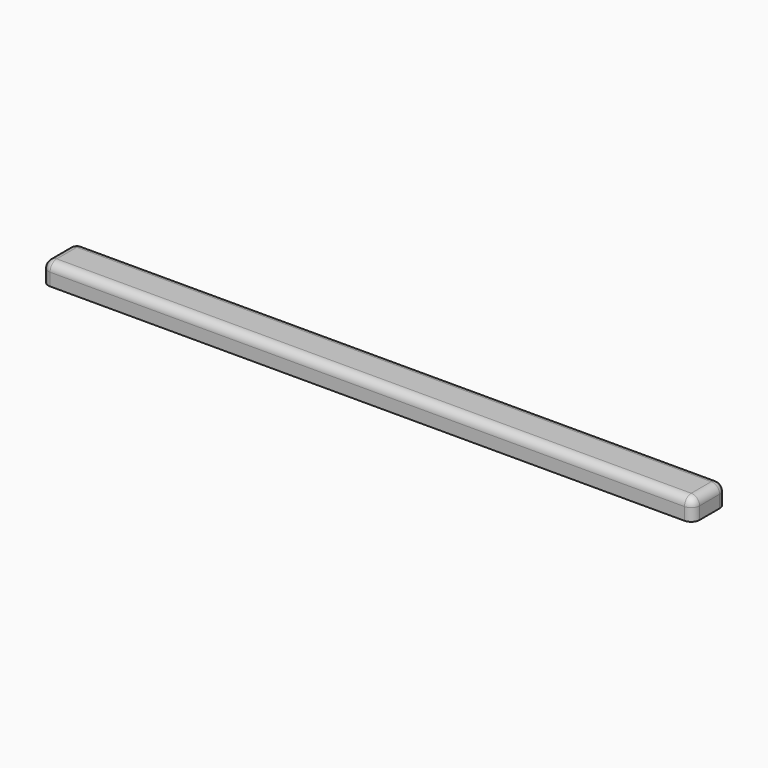
from build123d import *

# Parameters (mm, degrees)
F0_W         = 156
F0_H         = 10
F1_DEPTH     = 5
F2_R         = 2
F3_T1_DEPTH  = 8
F3_S5_W      = 2
F3_S5_H      = 2
F3_T6_DEPTH  = 2
F3_S11_W     = 2
F3_S11_H     = 2
F3_T12_DEPTH = 2
F3_S17_W     = 2
F3_S17_H     = 2
F3_T18_DEPTH = 2
F3_S23_W     = 2
F3_S23_H     = 2
F3_T24_DEPTH = 2


# Not quite as in the source:
# - a fillet or chamfer that OpenCascade refuses, or shapes differently, is made with other operations: its cross-section is extruded or revolved along the edge and cut away or added


with BuildPart() as f1:
    # F0 (on Top) → F1 (new body)
    with BuildSketch(Plane.XY):
        with Locations((-78, 5)):
            Rectangle(F0_W, F0_H)
    extrude(amount=F1_DEPTH)

    # F2
    f2_edges = [f1.edges().sort_by_distance(p)[0] for p in [
        (-78, 10, 5),
        (-156, 5, 5),
        (-78, 0, 5),
        (0, 5, 5),
    ]]
    fillet(f2_edges, radius=F2_R)

    # F3: fillet of radius 2 on 4 edges, made by hand

    # F3_s2 → F3_t1 (cut)
    with BuildSketch(Plane.XY.offset(-5)):
        with BuildLine():
            ThreePointArc((0, 8), (-0.5857864376, 9.4142135624), (-2, 10))
            Line((-2, 10), (0, 10))
            Line((0, 10), (0, 8))
        make_face()
        with BuildLine():
            ThreePointArc((-2, 0), (-0.5857864376, 0.5857864376), (0, 2))
            Line((0, 2), (0, 0))
            Line((0, 0), (-2, 0))
        make_face()
        with BuildLine():
            ThreePointArc((-154, 0), (-155.4142135624, 0.5857864376), (-156, 2))
            Line((-156, 2), (-156, 0))
            Line((-156, 0), (-154, 0))
        make_face()
        with BuildLine():
            ThreePointArc((-156, 8), (-155.4142135624, 9.4142135624), (-154, 10))
            Line((-154, 10), (-156, 10))
            Line((-156, 10), (-156, 8))
        make_face()
    extrude(amount=F3_T1_DEPTH, mode=Mode.SUBTRACT)


with BuildPart() as f3_tool4:
    # F3_s5 → F3_t6 (new body)
    with BuildSketch(Plane.YZ.offset(-154)):
        with Locations((9, 4)):
            Rectangle(F3_S5_W, F3_S5_H)
    extrude(amount=-F3_T6_DEPTH)

    # F3_s7 → F3_t8 (revolve, cut)
    with BuildSketch(Plane(origin=(-154, 8, 3), x_dir=(0, -0.7071067812, -0.7071067812), z_dir=(0, 0.7071067812, -0.7071067812))):
        with BuildLine():
            ThreePointArc((0, -2), (2, 0), (0, 2))
            Line((0, 2), (0, -2))
        make_face()
    revolve(axis=Axis((-154, 8, 3), (-1, 0, 0)), mode=Mode.SUBTRACT)


with BuildPart() as f1_1:
    add(f1.part)

    # F3_t3: cut F3_tool4
    add(f3_tool4.part, mode=Mode.SUBTRACT)


with BuildPart() as f3_tool10:
    # F3_s11 → F3_t12 (new body)
    with BuildSketch(Plane.XZ.offset(-2)):
        with Locations((-155, 4)):
            Rectangle(F3_S11_W, F3_S11_H)
    extrude(amount=F3_T12_DEPTH)

    # F3_s13 → F3_t14 (revolve, cut)
    with BuildSketch(Plane(origin=(-154, 2, 3), x_dir=(0.7071067812, 0, -0.7071067812), z_dir=(-0.7071067812, 0, -0.7071067812))):
        with BuildLine():
            ThreePointArc((0, -2), (2, 0), (0, 2))
            Line((0, 2), (0, -2))
        make_face()
    revolve(axis=Axis((-154, 2, 3), (0, -1, 0)), mode=Mode.SUBTRACT)


with BuildPart() as f1_2:
    add(f1_1.part)

    # F3_t9: cut F3_tool10
    add(f3_tool10.part, mode=Mode.SUBTRACT)


with BuildPart() as f3_tool16:
    # F3_s17 → F3_t18 (new body)
    with BuildSketch(Plane.XZ.offset(-2)):
        with Locations((-1, 4)):
            Rectangle(F3_S17_W, F3_S17_H)
    extrude(amount=F3_T18_DEPTH)

    # F3_s19 → F3_t20 (revolve, cut)
    with BuildSketch(Plane(origin=(-2, 2, 3), x_dir=(-0.7071067812, 0, -0.7071067812), z_dir=(-0.7071067812, 0, 0.7071067812))):
        with BuildLine():
            ThreePointArc((0, -2), (2, 0), (0, 2))
            Line((0, 2), (0, -2))
        make_face()
    revolve(axis=Axis((-2, 2, 3), (0, -1, 0)), mode=Mode.SUBTRACT)


with BuildPart() as f1_3:
    add(f1_2.part)

    # F3_t15: cut F3_tool16
    add(f3_tool16.part, mode=Mode.SUBTRACT)


with BuildPart() as f3_tool22:
    # F3_s23 → F3_t24 (new body)
    with BuildSketch(Plane.YZ.offset(-2)):
        with Locations((9, 4)):
            Rectangle(F3_S23_W, F3_S23_H)
    extrude(amount=F3_T24_DEPTH)

    # F3_s25 → F3_t26 (revolve, cut)
    with BuildSketch(Plane(origin=(-2, 8, 3), x_dir=(0, -0.7071067812, -0.7071067812), z_dir=(0, -0.7071067812, 0.7071067812))):
        with BuildLine():
            ThreePointArc((0, -2), (2, 0), (0, 2))
            Line((0, 2), (0, -2))
        make_face()
    revolve(axis=Axis((-2, 8, 3), (1, 0, 0)), mode=Mode.SUBTRACT)


with BuildPart() as f1_4:
    add(f1_3.part)

    # F3_t21: cut F3_tool22
    add(f3_tool22.part, mode=Mode.SUBTRACT)


solid = f1_4.part
